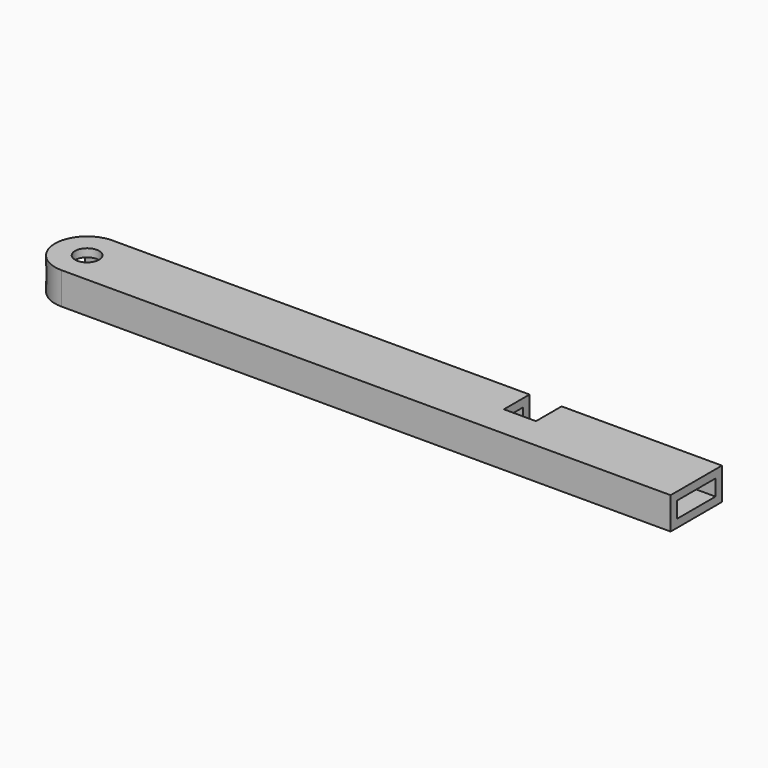
from build123d import *

# Parameters (mm, degrees)
F0_W          = 254
F0_H          = 25.4
F1_DEPTH      = 6.35
F2_R          = 12.69999
F3_R          = 4.7625
F4_DEPTH      = 12.701
F5_W          = 19.05
F5_H          = 6.35
F6_DEPTH      = 127.001
F6_DEPTH_BACK = 127.001
F7_W          = 12.7
F7_H          = 12.7
F8_DEPTH      = 12.701


# Not quite as in the source:
# - a fillet or chamfer is up to 0.001 mm smaller than in the source, because OpenCascade refuses the exact size


with BuildPart() as f1:
    # F0 (on Top) → F1 (new body, symmetric)
    with BuildSketch(Plane.XY):
        Rectangle(F0_W, F0_H)
    extrude(amount=F1_DEPTH, both=True)

    # F2 (radius 12.7 in the source; OpenCascade refuses exactly that, so slightly less here)
    f2_edges = [f1.edges().sort_by_distance(p)[0] for p in [
        (-127, 12.7, 0),
        (-127, -12.7, 0),
    ]]
    fillet(f2_edges, radius=F2_R)

    # F3 (on face) → F4 (cut, through all)
    with BuildSketch(Plane.XY.offset(6.35)):
        with Locations((-114.3, 0)):
            Circle(F3_R)
    extrude(amount=-F4_DEPTH, mode=Mode.SUBTRACT)

    # F5 (on Right) → F6 (cut, two sides)
    with BuildSketch(Plane.YZ) as f6_sk:
        Rectangle(F5_W, F5_H)
    extrude(amount=-F6_DEPTH, mode=Mode.SUBTRACT)
    extrude(f6_sk.sketch, amount=F6_DEPTH_BACK, mode=Mode.SUBTRACT)

    # F7 (on face) → F8 (cut, through all)
    with BuildSketch(Plane.XY.offset(6.35)):
        with Locations((57.15, 6.35)):
            Rectangle(F7_W, F7_H)
    extrude(amount=-F8_DEPTH, mode=Mode.SUBTRACT)


solid = f1.part
